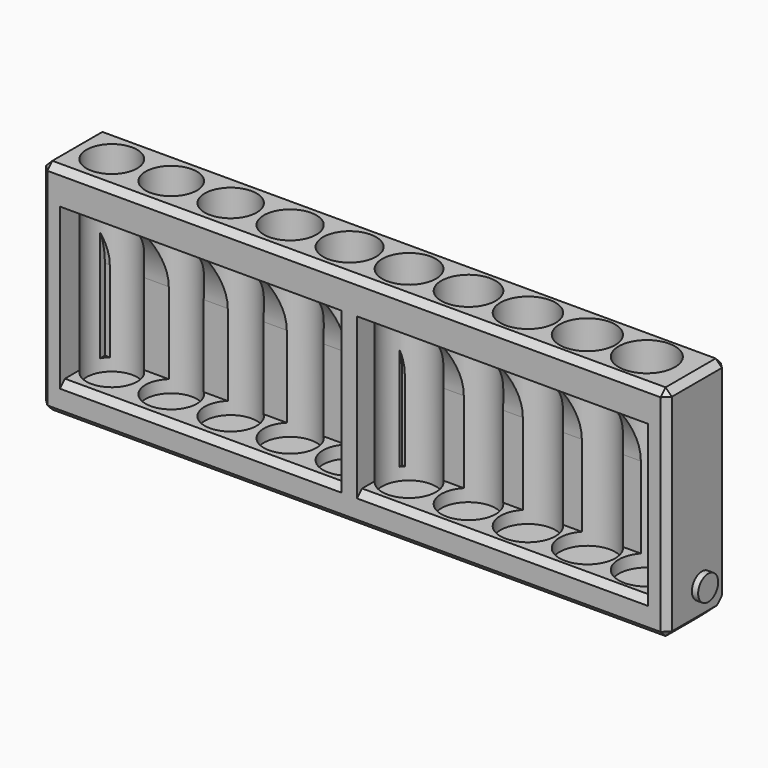
from build123d import *

# Parameters (mm, degrees)
F0_W          = 100
F0_H          = 12
F2_DEPTH      = 35
F3_START      = 3
F1_R          = 4.5
F1_R_2        = 4.45
F1_R_3        = 4.4
F1_R_4        = 4.35
F1_R_5        = 4.3
F1_R_6        = 4.25
F1_R_7        = 4.2
F1_R_8        = 4.15
F1_R_9        = 4.1
F1_R_10       = 4.05
F3_DEPTH      = 37
F5_START      = -3
F5_DEPTH      = 46.5
F6_START      = -52
F6_DEPTH      = 45
F7_SIZE       = 1
F8_R          = 2
F9_DEPTH      = 2
F9_DEPTH_BACK = 1
F10_START     = -99
F10_DEPTH     = 2
F11_T1_DEPTH  = 123


# Not quite as in the source:
# - a fillet or chamfer that OpenCascade refuses, or shapes differently, is made with other operations: its cross-section is extruded or revolved along the edge and cut away or added


with BuildPart() as f2:
    # F0 (on Top) → F2 (new body)
    with BuildSketch(Plane.XY):
        with Locations((-50, -6)):
            Rectangle(F0_W, F0_H)
    extrude(amount=F2_DEPTH)

    # F1 (on Top) → F3 (cut)
    with BuildSketch(Plane.XY.offset(F3_START)):
        with Locations((-8, -6)):
            Circle(F1_R)
        with Locations((-17.5, -6)):
            Circle(F1_R_2)
        with Locations((-27, -6)):
            Circle(F1_R_3)
        with Locations((-36.5, -6)):
            Circle(F1_R_4)
        with Locations((-46, -6)):
            Circle(F1_R_5)
        with Locations((-55.5, -6)):
            Circle(F1_R_6)
        with Locations((-65, -6)):
            Circle(F1_R_7)
        with Locations((-74.5, -6)):
            Circle(F1_R_8)
        with Locations((-84, -6)):
            Circle(F1_R_9)
        with Locations((-93.5, -6)):
            Circle(F1_R_10)
    extrude(amount=F3_DEPTH, mode=Mode.SUBTRACT)

    # F4 (on Right) → F5 (cut)
    with BuildSketch(Plane.YZ.offset(F5_START)):
        with BuildLine():
            Line((-13, 29.8321595662), (-13, 5))
            Line((-13, 5), (-3, 5))
            Line((-3, 5), (-3, 18))
            ThreePointArc((-3, 18), (-5.8348486101, 25.7459666924), (-13, 29.8321595662))
        make_face()
        with BuildLine():
            ThreePointArc((-15, 30), (-13.9964848766, 29.9579662735), (-13, 29.8321595662))
            Line((-13, 29.8321595662), (-13, 30))
            Line((-13, 30), (-15, 30))
        make_face()
    extrude(amount=-F5_DEPTH, mode=Mode.SUBTRACT)

    # F4 (on Right) → F6 (cut)
    with BuildSketch(Plane.YZ.offset(F6_START)):
        with BuildLine():
            Line((-13, 29.8321595662), (-13, 5))
            Line((-13, 5), (-3, 5))
            Line((-3, 5), (-3, 18))
            ThreePointArc((-3, 18), (-5.8348486101, 25.7459666924), (-13, 29.8321595662))
        make_face()
        with BuildLine():
            ThreePointArc((-15, 30), (-13.9964848766, 29.9579662735), (-13, 29.8321595662))
            Line((-13, 29.8321595662), (-13, 30))
            Line((-13, 30), (-15, 30))
        make_face()
    extrude(amount=-F6_DEPTH, mode=Mode.SUBTRACT)

    # F7
    f7_edges = [f2.edges().sort_by_distance(p)[0] for p in [
        (-50, -12, 35),
        (-100, -6, 35),
        (-50, 0, 35),
        (0, -6, 35),
        (0, -12, 17.5),
        (0, 0, 17.5),
        (0, -6, 0),
        (-50, -12, 0),
        (-100, -12, 17.5),
        (-74.5, -12, 5),
        (-26.25, -12, 5),
        (-100, -6, 0),
        (-100, 0, 17.5),
    ]]
    chamfer(f7_edges, length=F7_SIZE)

    # F8 (on Right) → F9 (join, two sides)
    with BuildSketch(Plane.YZ) as f9_sk:
        with Locations((-5, 5)):
            Circle(F8_R)
    extrude(amount=-F9_DEPTH)
    extrude(f9_sk.sketch, amount=F9_DEPTH_BACK)

    # F8 (on Right) → F10 (join)
    with BuildSketch(Plane.YZ.offset(F10_START)):
        with Locations((-5, 5)):
            Circle(F8_R)
    extrude(amount=-F10_DEPTH)

    # F11: fillet of radius 5 on 1 edges, made by hand

    # F11_s2 → F11_t1 (cut)
    with BuildSketch(Plane.YZ.offset(-111.5)):
        with BuildLine():
            ThreePointArc((0, 5), (-1.4644660941, 1.4644660941), (-5, 0))
            Line((-5, 0), (0, 0))
            Line((0, 0), (0, 5))
        make_face()
    extrude(amount=F11_T1_DEPTH, mode=Mode.SUBTRACT)


solid = f2.part
